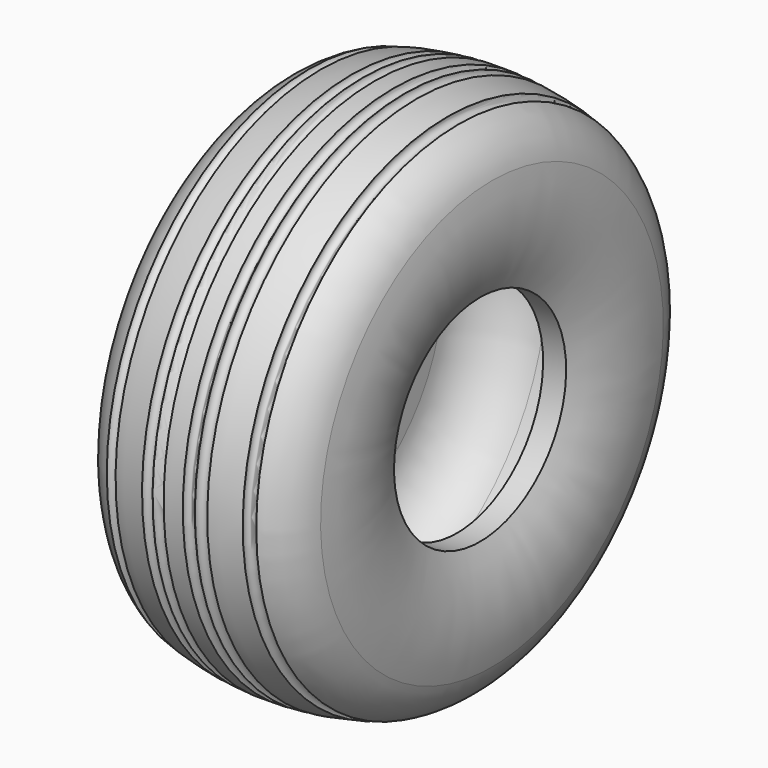
from build123d import *


# Not quite as in the source:
# - a fillet or chamfer that OpenCascade refuses, or shapes differently, is made with other operations: its cross-section is extruded or revolved along the edge and cut away or added


with BuildPart() as f1:
    # F0 (on Front) → F1 (revolve)
    with BuildSketch(Plane.XZ):
        with BuildLine():
            Line((3.048, 3.556), (3.81, 3.556))
            ThreePointArc((3.81, 3.556), (4.3534149407, 5.842), (3.81, 8.128))
            ThreePointArc((3.81, 8.128), (3.4597534805, 8.2535838272), (3.1045587191, 8.3644017117))
            ThreePointArc((3.1045587191, 8.3644017117), (2.8720142857, 8.2312629184), (2.736391587, 8.4623675168))
            ThreePointArc((2.736391587, 8.4623675168), (2.2275870119, 8.5704833446), (1.7133301198, 8.6486560815))
            ThreePointArc((1.7133301198, 8.6486560815), (1.50495, 8.4801907217), (1.3342616659, 8.6867538945))
            ThreePointArc((1.3342616659, 8.6867538945), (1.3336614225, 8.6868012342), (1.3330611759, 8.6868485333))
            ThreePointArc((1.3330611759, 8.6868485333), (1.1321142857, 8.5095826338), (0.9527055588, 8.7086187122))
            ThreePointArc((0.9527055588, 8.7086187122), (0.635, 8.7142975126), (0.3172944412, 8.7086187122))
            ThreePointArc((0.3172944412, 8.7086187122), (0.3174486034, 8.7041962294), (0.3175, 8.6997713591))
            ThreePointArc((0.3175, 8.6997713591), (0.1334651371, 8.5093810967), (-0.0630611759, 8.6868485333))
            ThreePointArc((-0.0630611759, 8.6868485333), (-0.0636614225, 8.6868012342), (-0.0642616659, 8.6867538945))
            ThreePointArc((-0.0642616659, 8.6867538945), (-0.0636905117, 8.6782533796), (-0.0635, 8.6697358284))
            ThreePointArc((-0.0635, 8.6697358284), (-0.2434439075, 8.4795285233), (-0.4433301198, 8.6486560815))
            ThreePointArc((-0.4433301198, 8.6486560815), (-0.9575870119, 8.5704833446), (-1.466391587, 8.4623675168))
            ThreePointArc((-1.466391587, 8.4623675168), (-1.4619786352, 8.4390461557), (-1.4605, 8.4153570514))
            ThreePointArc((-1.4605, 8.4153570514), (-1.6252870265, 8.2266003482), (-1.8345587191, 8.3644017117))
            ThreePointArc((-1.8345587191, 8.3644017117), (-2.1897534805, 8.2535838272), (-2.54, 8.128))
            ThreePointArc((-2.54, 8.128), (-3.0834149407, 5.842), (-2.54, 3.556))
            Line((-2.54, 3.556), (-1.778, 3.556))
            Line((-1.778, 3.556), (-1.778, 7.366))
            Line((-1.778, 7.366), (3.048, 7.366))
            Line((3.048, 7.366), (3.048, 3.556))
        make_face()
    revolve(axis=Axis((0, 0, 0), (1, 0, 0)))

    # F2: fillet of radius 1.905 on 4 edges, made by hand

    # F2_s1 → F2_t2 (revolve)
    with BuildSketch(Plane.XZ):
        with BuildLine():
            ThreePointArc((1.143, 7.366), (2.4900384182, 6.8080384182), (3.048, 5.461))
            Line((3.048, 5.461), (3.048, 7.366))
            Line((3.048, 7.366), (1.143, 7.366))
        make_face()
    revolve(axis=Axis((3.048, 0, 0), (1, 0, 0)))

    # F2_s3 → F2_t4 (revolve)
    with BuildSketch(Plane.XZ):
        with BuildLine():
            ThreePointArc((0.127, 7.366), (-1.2200384182, 6.8080384182), (-1.778, 5.461))
            Line((-1.778, 5.461), (-1.778, 7.366))
            Line((-1.778, 7.366), (0.127, 7.366))
        make_face()
    revolve(axis=Axis((-1.778, 0, 0), (1, 0, 0)))

    # F2_s5 → F2_t6 (revolve, cut)
    with BuildSketch(Plane.XZ):
        with BuildLine():
            ThreePointArc((4.201018724, 7.076957876), (3.8034754564, 7.849013142), (3.1045587191, 8.3644017117))
            ThreePointArc((3.1045587191, 8.3644017117), (3.4597534805, 8.2535838272), (3.81, 8.128))
            ThreePointArc((3.81, 8.128), (4.0346007172, 7.6133017817), (4.201018724, 7.076957876))
        make_face()
    revolve(axis=Axis((3.81, 0, 0), (1, 0, 0)), mode=Mode.SUBTRACT)

    # F2_s7 → F2_t8 (revolve, cut)
    with BuildSketch(Plane.XZ):
        with BuildLine():
            ThreePointArc((-2.931018724, 7.076957876), (-2.5334754564, 7.849013142), (-1.8345587191, 8.3644017117))
            ThreePointArc((-1.8345587191, 8.3644017117), (-2.1897534805, 8.2535838272), (-2.54, 8.128))
            ThreePointArc((-2.54, 8.128), (-2.7646007172, 7.6133017817), (-2.931018724, 7.076957876))
        make_face()
    revolve(axis=Axis((-2.54, 0, 0), (1, 0, 0)), mode=Mode.SUBTRACT)


solid = f1.part
